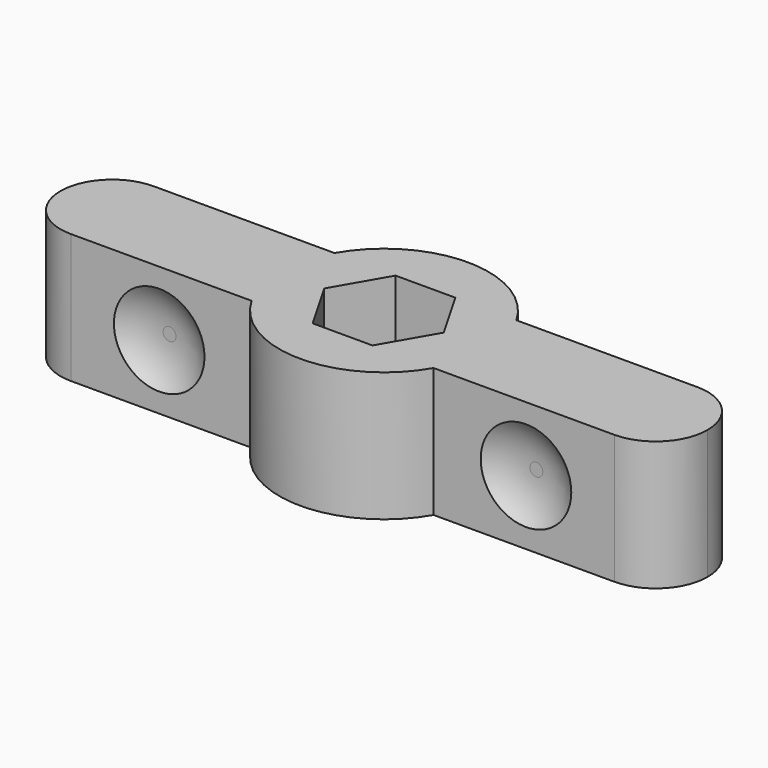
from build123d import *

# Parameters (mm, degrees)
F1_DEPTH = 10
F2_R     = 3.5
F4_DEPTH = 1
F3_R     = 3.5
F6_DEPTH = 1


# Not quite as in the source:
# - a fillet or chamfer that OpenCascade refuses, or shapes differently, is made with other operations: its cross-section is extruded or revolved along the edge and cut away or added


with BuildPart() as f1:
    # F0 (on Top) → F1 (new body)
    with BuildSketch(Plane.XY):
        with BuildLine():
            Line((-7.0290866446, 4), (-2.3094010768, 4))
            Line((-2.3094010768, 4), (2.3094010768, 4))
            Line((2.3094010768, 4), (7.0290866446, 4))
            ThreePointArc((7.0290866446, 4), (0, 8.087524903), (-7.0290866446, 4))
        make_face()
        with BuildLine():
            Line((-4.6188021535, 0), (-2.3094010768, 4))
            Line((-2.3094010768, 4), (-7.0290866446, 4))
            ThreePointArc((-7.0290866446, 4), (-8.087524903, 0), (-7.0290866446, -4))
            Line((-7.0290866446, -4), (-2.3094010768, -4))
            Line((-2.3094010768, -4), (-4.6188021535, 0))
        make_face()
        with BuildLine():
            Line((7.0290866446, 4), (2.3094010768, 4))
            Line((2.3094010768, 4), (4.6188021535, 0))
            Line((4.6188021535, 0), (2.3094010768, -4))
            Line((2.3094010768, -4), (7.0290866446, -4))
            ThreePointArc((7.0290866446, -4), (7.8184388576, -2.068833702), (8.087524903, 0))
            ThreePointArc((8.087524903, 0), (7.8184388576, 2.068833702), (7.0290866446, 4))
        make_face()
        with BuildLine():
            ThreePointArc((-7.0290866446, -4), (-8.087524903, 0), (-7.0290866446, 4))
            Line((-7.0290866446, 4), (-21, 4))
            ThreePointArc((-21, 4), (-23.8284271247, 2.8284271247), (-25, 0))
            ThreePointArc((-25, 0), (-23.8284271247, -2.8284271247), (-21, -4))
            Line((-21, -4), (-7.0290866446, -4))
        make_face()
        with BuildLine():
            Line((21, 4), (7.0290866446, 4))
            ThreePointArc((7.0290866446, 4), (7.8184388576, 2.068833702), (8.087524903, 0))
            ThreePointArc((8.087524903, 0), (7.8184388576, -2.068833702), (7.0290866446, -4))
            Line((7.0290866446, -4), (21, -4))
            ThreePointArc((21, -4), (23.8284271247, -2.8284271247), (25, 0))
            ThreePointArc((25, 0), (23.8284271247, 2.8284271247), (21, 4))
        make_face()
        with BuildLine():
            Line((2.3094010768, -4), (-2.3094010768, -4))
            Line((-2.3094010768, -4), (-7.0290866446, -4))
            ThreePointArc((-7.0290866446, -4), (0, -8.087524903), (7.0290866446, -4))
            Line((7.0290866446, -4), (2.3094010768, -4))
        make_face()
    extrude(amount=F1_DEPTH)

    # F2 (on face) → F4 (cut)
    with BuildSketch(Plane.XZ.offset(4)):
        with Locations((-14.1732281117, 5)):
            Circle(F2_R)
        with Locations((14.1732281117, 5)):
            Circle(F2_R)
    extrude(amount=-F4_DEPTH, mode=Mode.SUBTRACT)

    # F5: fillet of radius 5 on 2 edges, made by hand

    # F5_s1 → F5_t2 (revolve)
    with BuildSketch(Plane.XY.offset(5)):
        with BuildLine():
            ThreePointArc((-10.6732281117, -4), (-12.0920892816, -3.2565835097), (-13.6732281117, -3))
            Line((-13.6732281117, -3), (-10.6732281117, -3))
            Line((-10.6732281117, -3), (-10.6732281117, -4))
        make_face()
    revolve(axis=Axis((-14.1732281117, -3, 5), (0, -1, 0)))

    # F5_s3 → F5_t4 (revolve)
    with BuildSketch(Plane.XY.offset(5)):
        with BuildLine():
            ThreePointArc((17.6732281117, -4), (16.2543669417, -3.2565835097), (14.6732281117, -3))
            Line((14.6732281117, -3), (17.6732281117, -3))
            Line((17.6732281117, -3), (17.6732281117, -4))
        make_face()
    revolve(axis=Axis((14.1732281117, -3, 5), (0, -1, 0)))

    # F3 (on face) → F6 (cut)
    with BuildSketch(Plane(origin=(0, 4, 0), x_dir=(-1, 0, 0), z_dir=(0, 1, 0))):
        with Locations((13.4998997673, 5.0000185147)):
            Circle(F3_R)
        with Locations((-13.4998997673, 5.0000185147)):
            Circle(F3_R)
    extrude(amount=-F6_DEPTH, mode=Mode.SUBTRACT)

    # F7: fillet of radius 5 on 2 edges, made by hand

    # F7_s1 → F7_t2 (revolve)
    with BuildSketch(Plane.XY.offset(5.0000185147)):
        with BuildLine():
            ThreePointArc((9.9998997673, 4), (11.4187609373, 3.2565835097), (12.9998997673, 3))
            Line((12.9998997673, 3), (9.9998997673, 3))
            Line((9.9998997673, 3), (9.9998997673, 4))
        make_face()
    revolve(axis=Axis((13.4998997673, 3, 5.0000185147), (0, 1, 0)))

    # F7_s3 → F7_t4 (revolve)
    with BuildSketch(Plane.XY.offset(5.0000185147)):
        with BuildLine():
            ThreePointArc((-16.9998997673, 4), (-15.5810385974, 3.2565835097), (-13.9998997673, 3))
            Line((-13.9998997673, 3), (-16.9998997673, 3))
            Line((-16.9998997673, 3), (-16.9998997673, 4))
        make_face()
    revolve(axis=Axis((-13.4998997673, 3, 5.0000185147), (0, 1, 0)))


solid = f1.part
